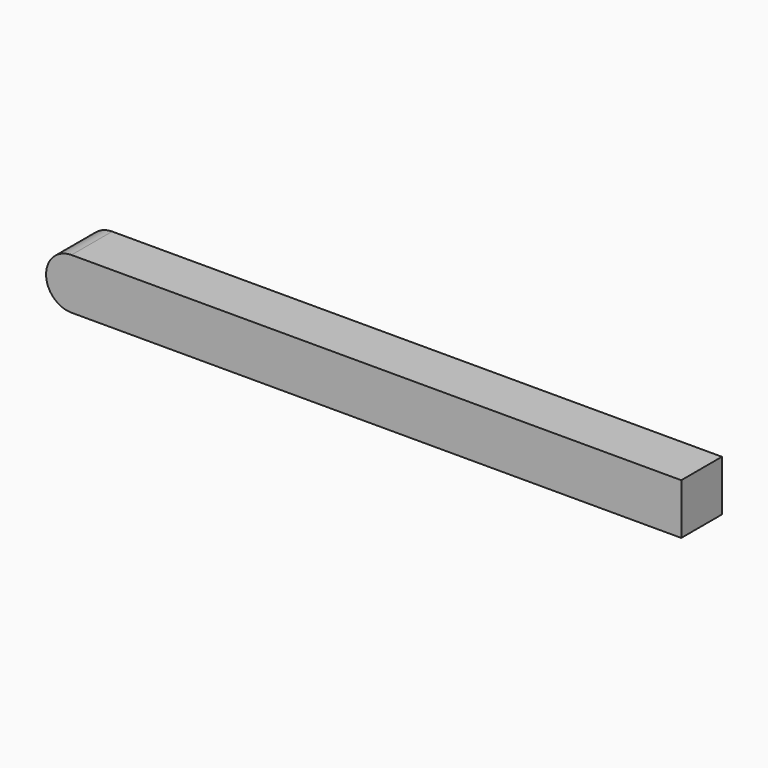
from build123d import *

# Parameters (mm, degrees)
F0_W     = 50
F0_H     = 4
F1_DEPTH = 4
F2_R     = 1.99999


# Not quite as in the source:
# - a fillet or chamfer is up to 0.001 mm smaller than in the source, because OpenCascade refuses the exact size


with BuildPart() as f1:
    # F0 (on Top) → F1 (new body)
    with BuildSketch(Plane.XY):
        with Locations((22.9771230485, -0.3226846457)):
            Rectangle(F0_W, F0_H)
    extrude(amount=F1_DEPTH)

    # F2 (radius 2 in the source; OpenCascade refuses exactly that, so slightly less here)
    f2_edges = [f1.edges().sort_by_distance(p)[0] for p in [
        (-2.022877, -0.322685, 0),
        (-2.022877, -0.322685, 4),
    ]]
    fillet(f2_edges, radius=F2_R)


solid = f1.part
